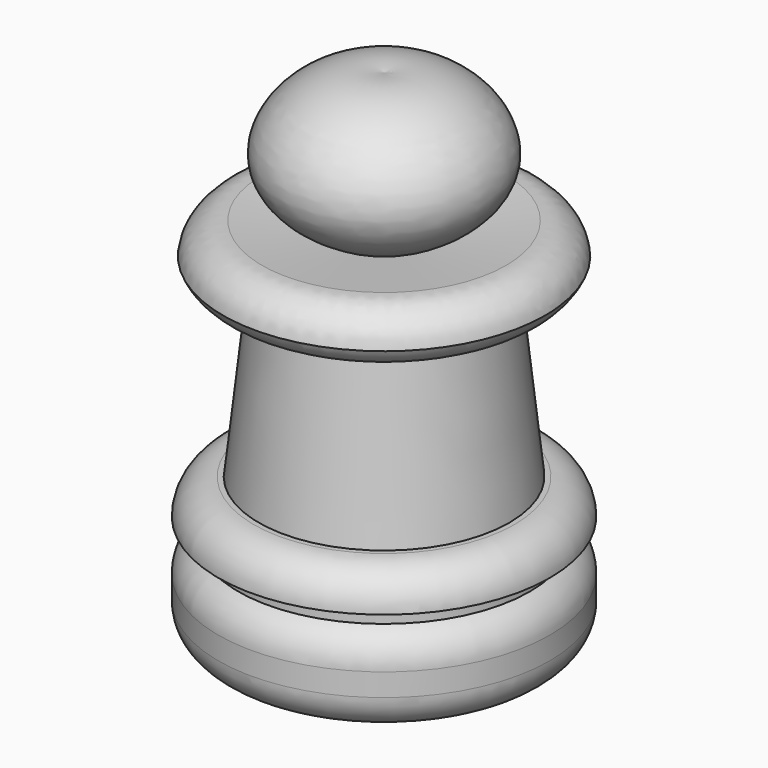
from build123d import *

# Parameters (mm, degrees)
F2_R = 5.08
F4_R = 5.08


# Not quite as in the source:
# - a fillet or chamfer that OpenCascade refuses, or shapes differently, is made with other operations: its cross-section is extruded or revolved along the edge and cut away or added


with BuildPart() as f1:
    # F0 (on Front) → F1 (revolve)
    with BuildSketch(Plane.XZ):
        with BuildLine():
            Line((0, 5.8903070167), (0, -65.7662302256))
            Line((0, -65.7662302256), (23.7847398967, -65.7662302256))
            Line((23.7847398967, -65.7662302256), (23.7847398967, -52.8708919883))
            Line((23.7847398967, -52.8708919883), (20.9191124886, -52.8708919883))
            Line((20.9191124886, -52.8708919883), (20.9191124886, -50.2918213606))
            Line((20.9191124886, -50.2918213606), (23.7847398967, -50.2918213606))
            Line((23.7847398967, -50.2918213606), (23.7847398967, -45.1336875558))
            Line((23.7847398967, -45.1336875558), (17.9734769241, -45.1336875558))
            Line((17.9734769241, -45.1336875558), (15.3330073302, -20.7826976066))
            Line((15.3330073302, -20.7826976066), (23.3936539069, -19.9086513261))
            Line((23.3936539069, -19.9086513261), (22.5615684061, -12.2349762668))
            Line((22.5615684061, -12.2349762668), (6.3811652362, -13.9894783497))
            add(Edge.make_bspline(
                [(6.3811652362, -13.9894783497), (15.9030873328, -9.7337774932), (17.1888817575, 1.0956468485), (5.7737650258, 7.1289198042), (0, 5.8903070167)],
                knots=[0, 0, 0, 0, 0.5061420739, 1, 1, 1, 1], degree=3))
        make_face()
    revolve(axis=Axis((0, 0, -29.9379616044), (0, 0, -1)))

    # F2
    f2_edges = [f1.edges().sort_by_distance(p)[0] for p in [
        (-22.561568, 0, -12.234976),
    ]]
    fillet(f2_edges, radius=F2_R)

    # F3: fillet of radius 5.08 on 1 edges, made by hand

    # F3_s1 → F3_t2 (revolve, cut)
    with BuildSketch(Plane.XZ):
        with BuildLine():
            ThreePointArc((23.1092012062, -17.2853720543), (21.462024993, -19.4047848063), (18.9647026754, -20.3888991962))
            Line((18.9647026754, -20.3888991962), (23.3936539069, -19.9086513261))
            Line((23.3936539069, -19.9086513261), (23.1092012062, -17.2853720543))
        make_face()
    revolve(axis=Axis((0, 0, -19.9086513261), (0, 0, -1)), mode=Mode.SUBTRACT)

    # F4
    f4_edges = [f1.edges().sort_by_distance(p)[0] for p in [
        (-23.78474, 0, -45.133688),
    ]]
    fillet(f4_edges, radius=F4_R)

    # F5: fillet of radius 5.08 on 1 edges, made by hand

    # F5_s1 → F5_t2 (revolve, cut)
    with BuildSketch(Plane.XZ):
        with BuildLine():
            ThreePointArc((23.7847398967, -50.2136875558), (23.3426841199, -50.2722502096), (22.8971957765, -50.2918213606))
            Line((22.8971957765, -50.2918213606), (23.7847398967, -50.2918213606))
            Line((23.7847398967, -50.2918213606), (23.7847398967, -50.2136875558))
        make_face()
    revolve(axis=Axis((0, 0, -50.2918213606), (0, 0, -1)), mode=Mode.SUBTRACT)

    # F6: fillet of radius 5.08 on 3 edges, made by hand

    # F6_s1 → F6_t2 (revolve, cut)
    with BuildSketch(Plane.XZ):
        with BuildLine():
            ThreePointArc((23.7847398967, -60.6862302256), (22.2968423451, -64.278332674), (18.7047398967, -65.7662302256))
            Line((18.7047398967, -65.7662302256), (18.7047398967, -65.8678302256))
            Line((18.7047398967, -65.8678302256), (23.8863398967, -65.8678302256))
            Line((23.8863398967, -65.8678302256), (23.8863398967, -60.6862302256))
            Line((23.8863398967, -60.6862302256), (23.7847398967, -60.6862302256))
        make_face()
    revolve(axis=Axis((0, 0, -65.7662302256), (0, 0, -1)), mode=Mode.SUBTRACT)

    # F6_s3 → F6_t4 (revolve, cut)
    with BuildSketch(Plane.XZ):
        with BuildLine():
            ThreePointArc((20.9191124886, -52.8708919883), (23.0091221268, -54.7449614249), (23.7847398967, -57.4428668377))
            Line((23.7847398967, -57.4428668377), (23.8863398967, -57.4428668377))
            Line((23.8863398967, -57.4428668377), (23.8863398967, -52.8708919883))
            Line((23.8863398967, -52.8708919883), (23.7847398967, -52.7692919883))
            ThreePointArc((23.7847398967, -52.7692919883), (22.3519261926, -52.7692919883), (20.9633999405, -52.7794524913))
            Line((20.9633999405, -52.7794524913), (20.9191124886, -52.8708919883))
        make_face()
    revolve(axis=Axis((0, 0, -52.8708919883), (0, 0, -1)), mode=Mode.SUBTRACT)


solid = f1.part
